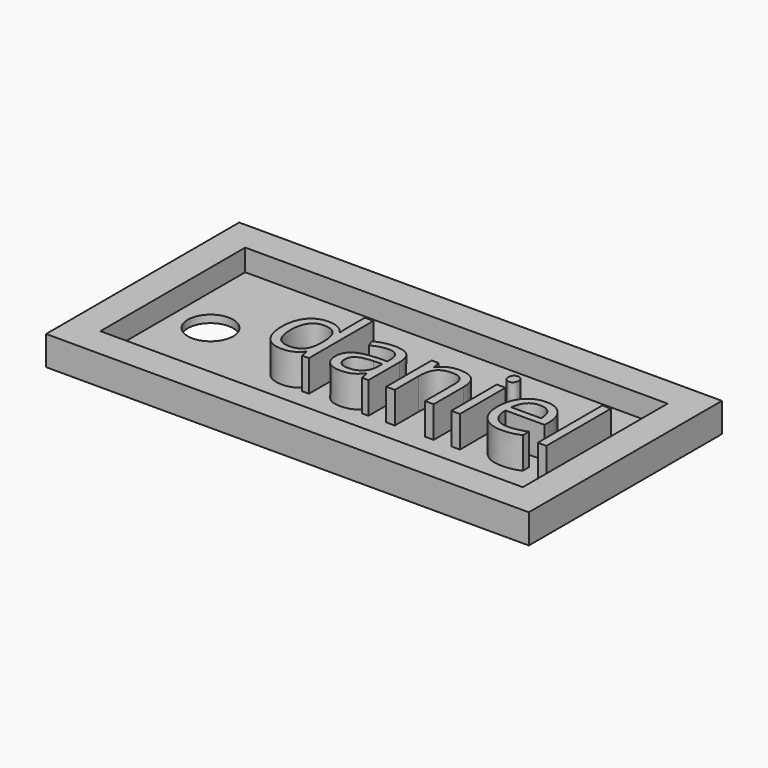
from build123d import *

# Parameters (mm, degrees)
F0_W         = 50.8
F0_H         = 25.4
F0_W_2       = 44.45
F0_H_2       = 19.05
F1_DEPTH     = 2.286
F0_R         = 2.38125
F1_FACE_W    = 50.8
F1_FACE_H    = 25.4
F1_FACE_W_2  = 44.45
F1_FACE_H_2  = 19.05
F2_DEPTH     = 0.79375
F3_TEXT_SIZE = 11.1723396306
F4_DEPTH     = 3.302


# Not quite as in the source:
# - Text() gives the source's letters only with a copy of the font that has no kerning and outlines rounded to 1/6400 em; it was checked with that copy


with BuildPart() as f1:
    # F0 (on Top) → F1 (new body)
    with BuildSketch(Plane.XY):
        with Locations((25.4, 12.7)):
            Rectangle(F0_W, F0_H)
        with Locations((25.4, 12.7)):
            Rectangle(F0_W_2, F0_H_2, mode=Mode.SUBTRACT)
    extrude(amount=F1_DEPTH)

    # F0 (on Top) + F1_face (on face) → F2 (join)
    with BuildSketch(Plane.XY):
        with Locations((25.4, 12.7)):
            Rectangle(F0_W_2, F0_H_2)
        with Locations((7.14375, 12.7)):
            Circle(F0_R, mode=Mode.SUBTRACT)
    with BuildSketch(Plane(origin=(25.4, 12.7, 2.286), x_dir=(1, 0, 0), z_dir=(0, 0, 1))):
        Rectangle(F1_FACE_W, F1_FACE_H)
        Rectangle(F1_FACE_W_2, F1_FACE_H_2, mode=Mode.SUBTRACT)
    extrude(amount=F2_DEPTH)

    # F3 (on face) → F4 (join)
    with BuildSketch(Plane.XY.offset(0.79375)):
        with Locations((14.8879121989, 8.6050014943)):
            Text('daniel', F3_TEXT_SIZE, font='Open Sans', text_align=(TextAlign.LEFT, TextAlign.BOTTOM))
    extrude(amount=F4_DEPTH)


solid = f1.part
